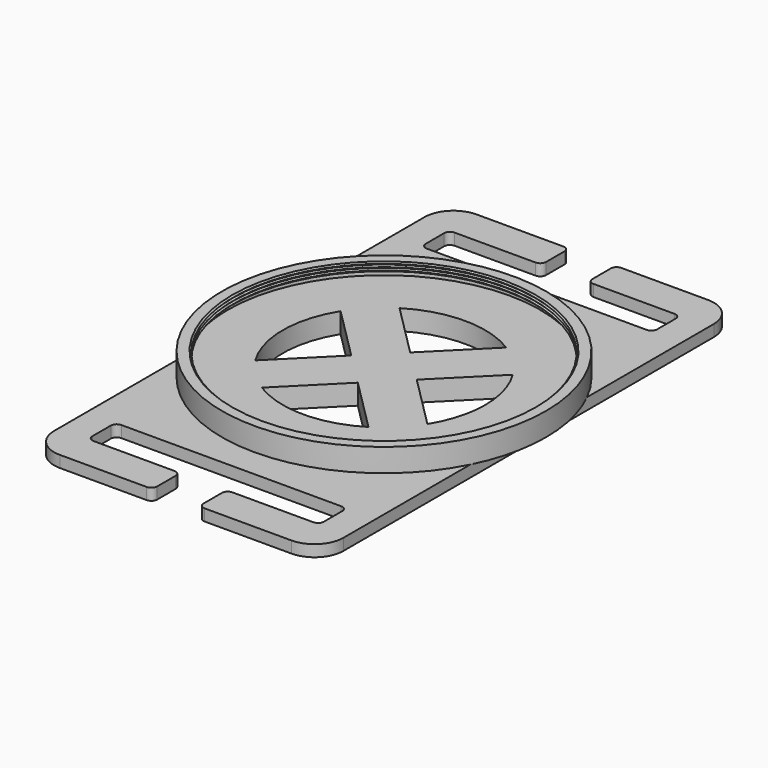
from build123d import *

# Parameters (mm, degrees)
F0_W      = 50
F0_H      = 90
F1_DEPTH  = 2
F2_R      = 28
F3_DEPTH  = 1.5
F4_R      = 28
F4_R_2    = 27
F5_DEPTH  = 1
F6_W      = 3
F6_H      = 70
F7_DEPTH  = 3
F8_DEPTH  = 3
F10_DEPTH = 25
F11_W     = 8
F11_H     = 6
F12_DEPTH = 25
F13_R     = 1
F14_R     = 1
F15_R     = 5
F18_SIZE  = 0.25
F19_R     = 28
F19_R_2   = 27.25
F19_R_3   = 26
F20_DEPTH = 0.5
F21_SIZE  = 0.24999
F22_R     = 28
F22_R_2   = 26.24999
F22_R_3   = 26
F23_DEPTH = 0.5
F24_SIZE  = 0.2499
F25_R     = 28
F25_R_2   = 26.2499
F25_R_3   = 26
F26_DEPTH = 0.5
F27_SIZE  = 0.249


# Not quite as in the source:
# - a fillet or chamfer is up to 0.001 mm smaller than in the source, because OpenCascade refuses the exact size


with BuildPart() as f1:
    # F0 (on Top) → F1 (new body)
    with BuildSketch(Plane.XY):
        Rectangle(F0_W, F0_H)
    extrude(amount=F1_DEPTH)

    # F2 (on face) → F3 (join)
    with BuildSketch(Plane.XY.offset(2)):
        Circle(F2_R)
    extrude(amount=F3_DEPTH)

    # F4 (on face) → F5 (join)
    with BuildSketch(Plane.XY.offset(3.5)):
        Circle(F4_R)
        Circle(F4_R_2, mode=Mode.SUBTRACT)
    extrude(amount=F5_DEPTH)

    # F6 (on face) → F7 (join)
    with BuildSketch(Plane(origin=(0, 0, 0), x_dir=(1, 0, 0), z_dir=(0, 0, -1))):
        with Locations((-23.5, 0)):
            Rectangle(F6_W, F6_H)
        with Locations((23.5, 0)):
            Rectangle(F6_W, F6_H)
    extrude(amount=F7_DEPTH)

    # F8 (cut, through all): faces of the model
    f8_faces = [f1.faces().sort_by_distance(p)[0] for p in [
        (-23.5, 0, -3),
        (23.5, 0, -3),
        (-23.5, 0, -3),
        (23.5, 0, -3),
    ]]
    extrude(f8_faces, amount=-F8_DEPTH, mode=Mode.SUBTRACT)

    # F9 (on face) → F10 (cut)
    with BuildSketch(Plane.XY.offset(3.5)):
        with BuildLine():
            Line((-5.6568542495, 0), (-14.8752109279, 9.2183566784))
            ThreePointArc((-14.8752109279, 9.2183566784), (-17.5, 0), (-14.8752109279, -9.2183566784))
            Line((-14.8752109279, -9.2183566784), (-5.6568542495, 0))
        make_face()
        with BuildLine():
            ThreePointArc((-9.2183566784, -14.8752109279), (0, -17.5), (9.2183566784, -14.8752109279))
            Line((9.2183566784, -14.8752109279), (0, -5.6568542495))
            Line((0, -5.6568542495), (-9.2183566784, -14.8752109279))
        make_face()
        with BuildLine():
            ThreePointArc((14.8752109279, -9.2183566784), (16.831015882, -4.7923798244), (17.5, 0))
            ThreePointArc((17.5, 0), (16.831015882, 4.7923798244), (14.8752109279, 9.2183566784))
            Line((14.8752109279, 9.2183566784), (5.6568542495, 0))
            Line((5.6568542495, 0), (14.8752109279, -9.2183566784))
        make_face()
        with BuildLine():
            Line((0, 5.6568542495), (9.2183566784, 14.8752109279))
            ThreePointArc((9.2183566784, 14.8752109279), (0, 17.5), (-9.2183566784, 14.8752109279))
            Line((-9.2183566784, 14.8752109279), (0, 5.6568542495))
        make_face()
    extrude(amount=-F10_DEPTH, mode=Mode.SUBTRACT)

    # F11 (on face) → F12 (cut)
    with BuildSketch(Plane(origin=(0, 0, 0), x_dir=(1, 0, 0), z_dir=(0, 0, -1))):
        with Locations((0, -42)):
            Rectangle(F11_W, F11_H)
        with BuildLine():
            Line((-4, -39), (4, -39))
            Line((4, -39), (19, -39))
            ThreePointArc((19, -39), (19.7071067812, -38.7071067812), (20, -38))
            Line((20, -38), (20, -34))
            ThreePointArc((20, -34), (19.7071067812, -33.2928932188), (19, -33))
            Line((19, -33), (-19, -33))
            ThreePointArc((-19, -33), (-19.7071067812, -33.2928932188), (-20, -34))
            Line((-20, -34), (-20, -38))
            ThreePointArc((-20, -38), (-19.7071067812, -38.7071067812), (-19, -39))
            Line((-19, -39), (-4, -39))
        make_face()
        with Locations((0, 42)):
            Rectangle(F11_W, F11_H)
        with BuildLine():
            ThreePointArc((20, 38), (19.7071067812, 38.7071067812), (19, 39))
            Line((19, 39), (4, 39))
            Line((4, 39), (-4, 39))
            Line((-4, 39), (-19, 39))
            ThreePointArc((-19, 39), (-19.7071067812, 38.7071067812), (-20, 38))
            Line((-20, 38), (-20, 34))
            ThreePointArc((-20, 34), (-19.7071067812, 33.2928932188), (-19, 33))
            Line((-19, 33), (19, 33))
            ThreePointArc((19, 33), (19.7071067812, 33.2928932188), (20, 34))
            Line((20, 34), (20, 38))
        make_face()
    extrude(amount=-F12_DEPTH, mode=Mode.SUBTRACT)

    # F13
    f13_edges = [f1.edges().sort_by_distance(p)[0] for p in [
        (-4, -45, 1),
        (-4, -39, 1),
        (4, -45, 1),
        (4, -39, 1),
    ]]
    fillet(f13_edges, radius=F13_R)

    # F14
    f14_edges = [f1.edges().sort_by_distance(p)[0] for p in [
        (4, 45, 1),
        (4, 39, 1),
        (-4, 45, 1),
        (-4, 39, 1),
    ]]
    fillet(f14_edges, radius=F14_R)

    # F15
    f15_edges = [f1.edges().sort_by_distance(p)[0] for p in [
        (25, -45, 1),
        (25, 45, 1),
        (-25, 45, 1),
        (-25, -45, 1),
    ]]
    fillet(f15_edges, radius=F15_R)


with BuildPart() as f16_1:
    # F16: copy of F1
    add(f1.part.moved(Location((72.1, 0, 0))))


with BuildPart() as f1_1:
    add(f1.part)

    # F18
    f18_edges = [f1_1.edges().sort_by_distance(p)[0] for p in [
        (-27, 0, 4.5),
    ]]
    chamfer(f18_edges, length=F18_SIZE)

    # F19 (on face) → F20 (join)
    with BuildSketch(Plane.XY.offset(4.5)):
        Circle(F19_R)
        Circle(F19_R_2, mode=Mode.SUBTRACT)
        Circle(F19_R_2)
        Circle(F19_R_3, mode=Mode.SUBTRACT)
    extrude(amount=F20_DEPTH)

    # F21 (size 0.25 in the source; OpenCascade refuses exactly that, so slightly less here)
    f21_edges = [f1_1.edges().sort_by_distance(p)[0] for p in [
        (-26, 0, 4.5),
        (-26, 0, 5),
    ]]
    chamfer(f21_edges, length=F21_SIZE)

    # F22 (on face) → F23 (join)
    with BuildSketch(Plane.XY.offset(5)):
        Circle(F22_R)
        Circle(F22_R_2, mode=Mode.SUBTRACT)
        Circle(F22_R_2)
        Circle(F22_R_3, mode=Mode.SUBTRACT)
    extrude(amount=F23_DEPTH)

    # F24 (size 0.25 in the source; OpenCascade refuses exactly that, so slightly less here)
    f24_edges = [f1_1.edges().sort_by_distance(p)[0] for p in [
        (-26, 0, 5),
        (-26, 0, 5.5),
    ]]
    chamfer(f24_edges, length=F24_SIZE)

    # F25 (on face) → F26 (join)
    with BuildSketch(Plane.XY.offset(5.5)):
        Circle(F25_R)
        Circle(F25_R_2, mode=Mode.SUBTRACT)
        Circle(F25_R_2)
        Circle(F25_R_3, mode=Mode.SUBTRACT)
    extrude(amount=F26_DEPTH)

    # F27 (size 0.25 in the source; OpenCascade refuses exactly that, so slightly less here)
    f27_edges = [f1_1.edges().sort_by_distance(p)[0] for p in [
        (-26, 0, 6),
        (-26, 0, 5.5),
    ]]
    chamfer(f27_edges, length=F27_SIZE)


solid = f1_1.part
